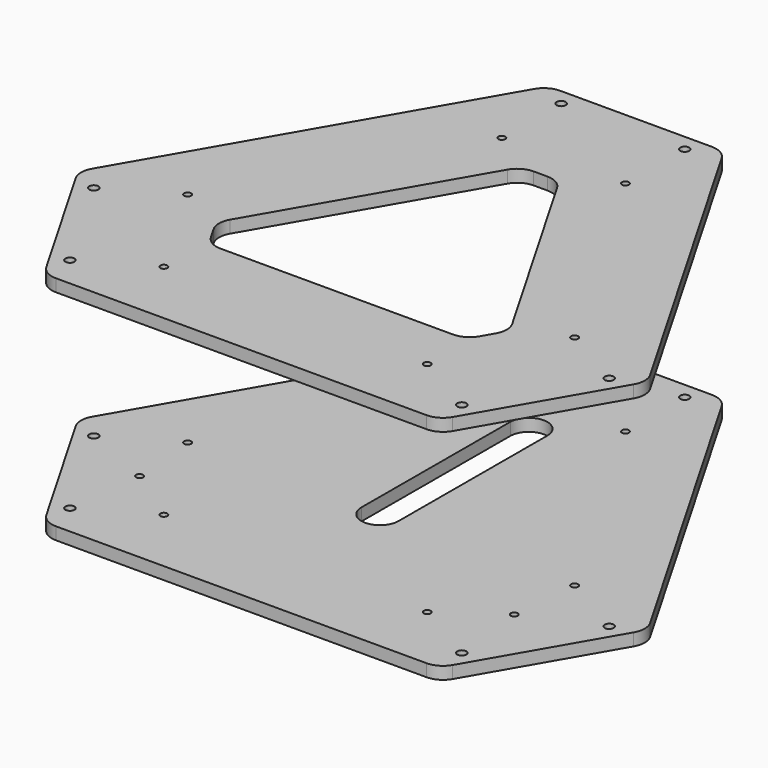
from build123d import *

# Parameters (mm, degrees)
F0_R     = 2.2
F0_R_2   = 1.7
F1_DEPTH = 6
F3_R     = 2.2
F3_R_2   = 1.7
F4_DEPTH = 6
F5_R     = 10
F5_2_R   = 10


# Not quite as in the source:
# - a feature names something its author has since deleted; it is built from what else it names


with BuildPart() as f1:
    # F0 (on Top) → F1 (new body)
    with BuildSketch(Plane.XY):
        Polygon((-42.617, 135.14210956), (-138.345, -30.6636501469), (-95.728, -104.4784594131), (95.728, -104.4784594131), (138.345, -30.6636501469), (42.617, 135.14210956), align=None)
        with Locations((-95.1082967697, -89.5518168935)):
            Circle(F0_R, mode=Mode.SUBTRACT)
        with Locations((-63.9313822335, -71.5518168935)):
            Circle(F0_R_2, mode=Mode.SUBTRACT)
        with Locations((-125.1082967697, -37.5902926665)):
            Circle(F0_R, mode=Mode.SUBTRACT)
        with Locations((-93.9313822335, -19.5902926665)):
            Circle(F0_R_2, mode=Mode.SUBTRACT)
        Polygon((71.372368774, -30.6636501469), (62.241684387, -46.4784594131), (-62.241684387, -46.4784594131), (-71.372368774, -30.6636501469), (-9.130684387, 77.14210956), (9.130684387, 77.14210956), align=None, mode=Mode.SUBTRACT)
        with Locations((63.9313822335, -71.5518168935)):
            Circle(F0_R_2, mode=Mode.SUBTRACT)
        with Locations((95.1082967697, -89.5518168935)):
            Circle(F0_R, mode=Mode.SUBTRACT)
        with Locations((93.9313822335, -19.5902926665)):
            Circle(F0_R_2, mode=Mode.SUBTRACT)
        with Locations((125.1082967697, -37.5902926665)):
            Circle(F0_R, mode=Mode.SUBTRACT)
        with Locations((-30, 91.14210956)):
            Circle(F0_R_2, mode=Mode.SUBTRACT)
        with Locations((-30, 127.14210956)):
            Circle(F0_R, mode=Mode.SUBTRACT)
        with Locations((30, 91.14210956)):
            Circle(F0_R_2, mode=Mode.SUBTRACT)
        with Locations((30, 127.14210956)):
            Circle(F0_R, mode=Mode.SUBTRACT)
    extrude(amount=F1_DEPTH)

    # F5
    f5_edges = [f1.edges().sort_by_distance(p)[0] for p in [
        (-95.728, -104.478459, 3),
        (-138.345, -30.66365, 3),
        (95.728, -104.478459, 3),
        (138.345, -30.66365, 3),
        (-42.617, 135.14211, 3),
        (42.617, 135.14211, 3),
        (-71.372369, -30.66365, 3),
        (-62.241684, -46.478459, 3),
        (-9.130684, 77.14211, 3),
        (9.130684, 77.14211, 3),
        (71.372369, -30.66365, 3),
        (62.241684, -46.478459, 3),
    ]]
    fillet(f5_edges, radius=F5_R)


with BuildPart() as f4:
    # F3 (on offset) → F4 (new body)
    with BuildSketch(Plane(origin=(0, 0, -100), x_dir=(1, 0, 0), z_dir=(0, 0, -1))):
        Polygon((95.728, 104.4784594131), (-95.728, 104.4784594131), (-138.345, 30.6636501469), (-42.617, -135.14210956), (42.617, -135.14210956), (138.345, 30.6636501469), align=None)
        with Locations((-30, -127.14210956)):
            Circle(F3_R, mode=Mode.SUBTRACT)
        with Locations((-30, -91.14210956)):
            Circle(F3_R_2, mode=Mode.SUBTRACT)
        with Locations((0, -105)):
            Circle(F3_R_2, mode=Mode.SUBTRACT)
        with BuildLine():
            Line((8.7580333745, 20.0241934108), (8.9999674821, -69.9754814103))
            ThreePointArc((8.9999674821, -69.9754814103), (0.0241934108, -78.9996423031), (-8.9999674821, -70.0238682318))
            Line((-8.9999674821, -70.0238682318), (-9.2419015897, 19.9758065892))
            ThreePointArc((-9.2419015897, 19.9758065892), (-0.2661275183, 28.9999674821), (8.7580333745, 20.0241934108))
        make_face(mode=Mode.SUBTRACT)
        with Locations((30, -127.14210956)):
            Circle(F3_R, mode=Mode.SUBTRACT)
        with Locations((30, -91.14210956)):
            Circle(F3_R_2, mode=Mode.SUBTRACT)
        with Locations((-125.1082967697, 37.5902926665)):
            Circle(F3_R, mode=Mode.SUBTRACT)
        with Locations((-93.9313822335, 19.5902926665)):
            Circle(F3_R_2, mode=Mode.SUBTRACT)
        with Locations((-90.9326673974, 52.5)):
            Circle(F3_R_2, mode=Mode.SUBTRACT)
        with Locations((-95.1082967697, 89.5518168935)):
            Circle(F3_R, mode=Mode.SUBTRACT)
        with Locations((-63.9313822335, 71.5518168935)):
            Circle(F3_R_2, mode=Mode.SUBTRACT)
        with Locations((93.9313822335, 19.5902926665)):
            Circle(F3_R_2, mode=Mode.SUBTRACT)
        with Locations((125.1082967697, 37.5902926665)):
            Circle(F3_R, mode=Mode.SUBTRACT)
        with Locations((63.9313822335, 71.5518168935)):
            Circle(F3_R_2, mode=Mode.SUBTRACT)
        with Locations((90.9326673974, 52.5)):
            Circle(F3_R_2, mode=Mode.SUBTRACT)
        with Locations((95.1082967697, 89.5518168935)):
            Circle(F3_R, mode=Mode.SUBTRACT)
    extrude(amount=F4_DEPTH)

    # F5#2
    f5_2_edges = [f4.edges().sort_by_distance(p)[0] for p in [
        (95.728, -104.478459, -103),
        (138.345, -30.66365, -103),
        (-95.728, -104.478459, -103),
        (-138.345, -30.66365, -103),
        (-42.617, 135.14211, -103),
        (42.617, 135.14211, -103),
    ]]
    fillet(f5_2_edges, radius=F5_2_R)


solid = Compound([f1.part, f4.part])
